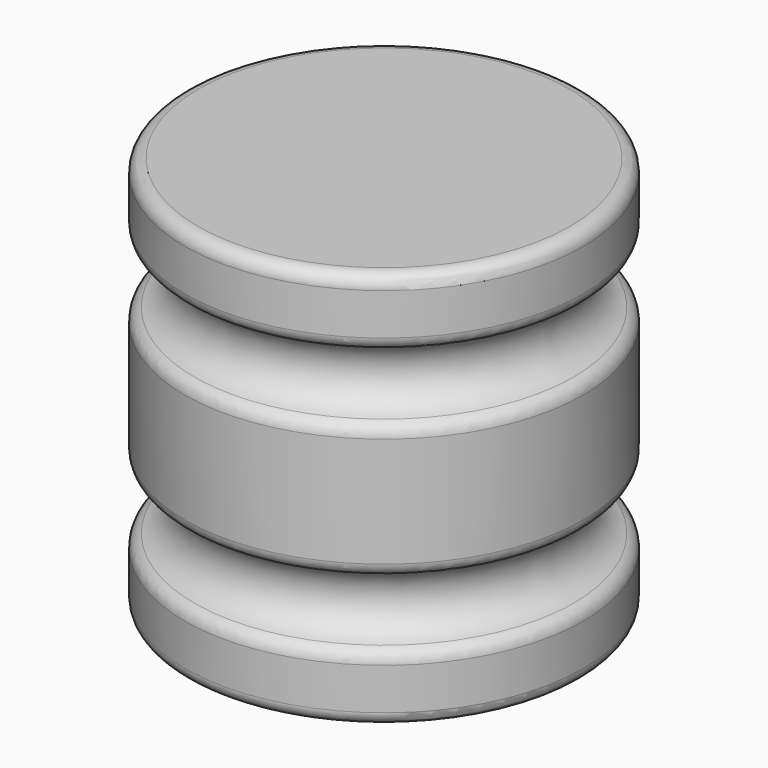
from build123d import *

# Parameters (mm, degrees)
F2_R = 2.54


with BuildPart() as f1:
    # F0 (on Front) → F1 (revolve)
    with BuildSketch(Plane.XZ):
        with BuildLine():
            Line((-38.1, 0), (0, 0))
            Line((0, 0), (0, 12.7))
            ThreePointArc((0, 12.7), (-6.35, 19.05), (0, 25.4))
            Line((0, 25.4), (0, 50.8))
            ThreePointArc((0, 50.8), (-6.35, 57.15), (0, 63.5))
            Line((0, 63.5), (0, 76.2))
            Line((0, 76.2), (-38.1, 76.2))
            Line((-38.1, 76.2), (-38.1, 0))
        make_face()
    revolve(axis=Axis((-38.1, 0, 38.1), (0, 0, 1)))

    # F2
    f2_edges = [f1.edges().sort_by_distance(p)[0] for p in [
        (-76.2, 0, 76.2),
        (-76.2, 0, 63.5),
        (-76.2, 0, 25.4),
        (-76.2, 0, 0),
        (-76.2, 0, 12.7),
        (0, 0, 6.35),
        (-76.2, 0, 50.8),
    ]]
    fillet(f2_edges, radius=F2_R)


solid = f1.part
